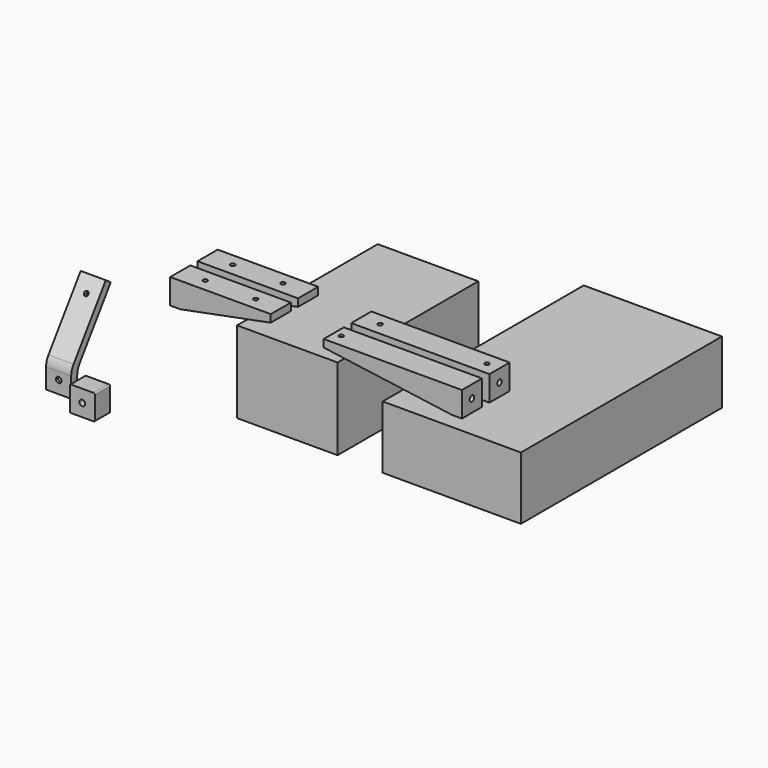
from build123d import *

# Parameters (mm, degrees)
F1_DEPTH   = 20
F3_R       = 1.75
F4_DEPTH   = 25
F5_R       = 3.5
F5_R_2     = 1.75
F6_DEPTH   = 3
F2_R       = 2.25
F7_DEPTH   = 25
F2_R_2     = 4
F8_DEPTH   = 4
F9_R       = 13
F10_W      = 80
F10_H      = 140
F11_DEPTH  = 65
F12_W      = 110
F12_H      = 200
F13_DEPTH  = 50
F15_DEPTH  = 20
F16_R      = 2.25
F17_DEPTH  = 122.8202211986
F18_DEPTH  = 4
F20_W      = 73.3484832836
F20_H      = 4
F22_R      = 1.75
F23_DEPTH  = 6.001
F22_R_2    = 3
F24_DEPTH  = 3
F26_DEPTH  = 20
F27_R      = 2.25
F28_DEPTH  = 4
F29_DEPTH  = 8.001
F31_W      = 102.9563014099
F31_H      = 4
F34_R      = 3
F34_R_2    = 1.75
F35_R      = 3
F35_R_2    = 1.75
F36_DEPTH  = 3
F36_FACE_R = 1.75
F37_DEPTH  = 9.6879868636
F38_DEPTH  = 3
F40_W      = 20
F40_H      = 20
F40_R      = 2.25
F41_DEPTH  = 15
F42_R      = 1


with BuildPart() as f1:
    # F0 (on Right) → F1 (new body)
    with BuildSketch(Plane.YZ):
        Polygon((0, 20), (0, 0), (6, 0), (6, 18.1082072667), (39.3294984468, 65.7076640392), (34.4145861811, 69.1491226573), align=None)
    extrude(amount=F1_DEPTH)

    # F3 (on face) → F4 (cut)
    with BuildSketch(Plane(origin=(0, -9.3969262079, 6.5797985667), x_dir=(1, 0, 0), z_dir=(0, -0.8191520443, 0.5735764364))):
        with Locations((10, 64.3830408858)):
            Circle(F3_R)
    extrude(amount=-F4_DEPTH, mode=Mode.SUBTRACT)

    # F5 (on face) → F6 (cut)
    with BuildSketch(Plane(origin=(0, -4.4820139421, 3.1383399486), x_dir=(-1, 0, 0), z_dir=(0, 0.8191520443, -0.5735764364))):
        with Locations((-10, 64.3830408858)):
            Circle(F5_R)
        with Locations((-10, 64.3830408858)):
            Circle(F5_R_2, mode=Mode.SUBTRACT)
    extrude(amount=-F6_DEPTH, mode=Mode.SUBTRACT)

    # F2 (on face) → F7 (cut)
    with BuildSketch(Plane(origin=(0, 6, 0), x_dir=(-1, 0, 0), z_dir=(0, 1, 0))):
        with Locations((-10, 10)):
            Circle(F2_R)
    extrude(amount=-F7_DEPTH, mode=Mode.SUBTRACT)

    # F2 (on face) → F8 (cut)
    with BuildSketch(Plane(origin=(0, 6, 0), x_dir=(-1, 0, 0), z_dir=(0, 1, 0))):
        with Locations((-10, 10)):
            Circle(F2_R_2)
        with Locations((-10, 10)):
            Circle(F2_R, mode=Mode.SUBTRACT)
    extrude(amount=-F8_DEPTH, mode=Mode.SUBTRACT)

    # F9
    f9_edges = [f1.edges().sort_by_distance(p)[0] for p in [
        (10, 6, 18.108207),
        (10, 0, 20),
    ]]
    fillet(f9_edges, radius=F9_R)


with BuildPart() as f11:
    # F10 (on Top) → F11 (new body)
    with BuildSketch(Plane.XY):
        with Locations((156.6803222895, 114.1342443228)):
            Rectangle(F10_W, F10_H)
    extrude(amount=F11_DEPTH)


with BuildPart() as f13:
    # F12 (on Top) → F13 (new body)
    with BuildSketch(Plane.XY):
        with Locations((288.3580553532, 143.2215481997)):
            Rectangle(F12_W, F12_H)
    extrude(amount=F13_DEPTH)


with BuildPart() as f15:
    # F14 (on Front) → F15 (new body)
    with BuildSketch(Plane.XZ):
        Polygon((114.8192211986, 124.3457761407), (114.8192211986, 104.3457761407), (122.8192211986, 104.3457761407), (122.8192211986, 118.3457761407), (194.8192211986, 118.3457761407), (194.8192211986, 124.3457761407), align=None)
    extrude(amount=F15_DEPTH)

    # F16 (on face) → F17 (cut, through all)
    with BuildSketch(Plane.YZ.offset(122.8192211986)):
        with Locations((-10, 114.3457761407)):
            Circle(F16_R)
    extrude(amount=-F17_DEPTH, mode=Mode.SUBTRACT)

    # F16 (on face) → F18 (cut)
    with BuildSketch(Plane.YZ.offset(122.8192211986)):
        with BuildLine():
            ThreePointArc((-10, 118.3457761407), (-12.8284271247, 111.5173490159), (-6, 114.3457761407))
            ThreePointArc((-6, 114.3457761407), (-7.1715728753, 117.1742032654), (-10, 118.3457761407))
        make_face()
        with Locations((-10, 114.3457761407)):
            Circle(F16_R, mode=Mode.SUBTRACT)
    extrude(amount=-F18_DEPTH, mode=Mode.SUBTRACT)

    # F20 (on 3pt) → F21 (join, up to the next surface of F15)
    with BuildSketch(Plane(origin=(-15.0758317834, 0, 77.532849172), x_dir=(0.9816153897, 0, 0.1908696591), z_dir=(-0.1908696591, 0, 0.9816153897))):
        with Locations((177.1519220381, -18)):
            Rectangle(F20_W, F20_H)
        with Locations((177.1519220381, -2)):
            Rectangle(F20_W, F20_H)
    extrude(until=Until.NEXT)

    # F22 (on face) → F23 (cut, through all)
    with BuildSketch(Plane(origin=(0, 0, 118.3457761407), x_dir=(1, 0, 0), z_dir=(0, 0, -1))):
        with Locations((134.8192211986, 10)):
            Circle(F22_R)
        with Locations((174.8192211986, 10)):
            Circle(F22_R)
    extrude(amount=-F23_DEPTH, mode=Mode.SUBTRACT)

    # F22 (on face) → F24 (cut)
    with BuildSketch(Plane(origin=(0, 0, 118.3457761407), x_dir=(1, 0, 0), z_dir=(0, 0, -1))):
        with Locations((134.8192211986, 10)):
            Circle(F22_R_2)
        with Locations((134.8192211986, 10)):
            Circle(F22_R, mode=Mode.SUBTRACT)
        with Locations((174.8192211986, 10)):
            Circle(F22_R_2)
        with Locations((174.8192211986, 10)):
            Circle(F22_R, mode=Mode.SUBTRACT)
    extrude(amount=-F24_DEPTH, mode=Mode.SUBTRACT)


with BuildPart() as f26:
    # F25 (on Front) → F26 (new body)
    with BuildSketch(Plane.XZ):
        Polygon((338.9809150696, 114.6587892771), (338.9809150696, 100.6587892771), (346.9809150696, 100.6587892771), (346.9809150696, 120.6587892771), (236.9809150696, 120.6587892771), (236.9809150696, 114.6587892771), align=None)
    extrude(amount=F26_DEPTH)

    # F27 (on face) → F28 (cut)
    with BuildSketch(Plane(origin=(338.9809150696, 0, 0), x_dir=(0, -1, 0), z_dir=(-1, 0, 0))):
        with BuildLine():
            ThreePointArc((10, 114.6587892771), (7.1715728753, 107.8303621523), (14, 110.6587892771))
            ThreePointArc((14, 110.6587892771), (12.8284271247, 113.4872164018), (10, 114.6587892771))
        make_face()
        with Locations((10, 110.6587892771)):
            Circle(F27_R, mode=Mode.SUBTRACT)
    extrude(amount=-F28_DEPTH, mode=Mode.SUBTRACT)

    # F29 (cut, through all): a face of the model
    f29_faces = [f26.faces().sort_by_distance(p)[0] for p in [
        (338.9809150696, -10, 110.6587892771),
    ]]
    extrude(f29_faces, amount=-F29_DEPTH, mode=Mode.SUBTRACT)

    # F31 (on 3pt) → F32 (join, up to the next surface of F26)
    with BuildSketch(Plane(origin=(19.8283972114, 0, 144.4640368262), x_dir=(0.9907115796, 0, -0.1359800207), z_dir=(0.1359800207, 0, 0.9907115796))):
        with Locations((270.6665828668, -18)):
            Rectangle(F31_W, F31_H)
        with Locations((270.6665828668, -2)):
            Rectangle(F31_W, F31_H)
    extrude(until=Until.NEXT)


with BuildPart() as f33_1:
    # F33: copy of F26
    add(f26.part.moved(Location((0, 27.4, 0))))


with BuildPart() as f36_tool:
    # F34 (on face) + F35 (on face) → F36 (new body)
    with BuildSketch(Plane(origin=(0, 0, 114.6587892771), x_dir=(1, 0, 0), z_dir=(0, 0, -1))):
        with Locations((242.9809150696, 10)):
            Circle(F34_R)
        with Locations((242.9809150696, 10)):
            Circle(F34_R_2, mode=Mode.SUBTRACT)
    with BuildSketch(Plane(origin=(0, 0, 114.6587892771), x_dir=(1, 0, 0), z_dir=(0, 0, -1))):
        with Locations((251.9809150696, -17.4)):
            Circle(F35_R)
        with Locations((251.9809150696, -17.4)):
            Circle(F35_R_2, mode=Mode.SUBTRACT)
        with BuildLine():
            Line((338.9809150696, -17.4), (338.9809150696, -15.1639320225))
            ThreePointArc((338.9809150696, -15.1639320225), (333.9809150696, -17.4), (338.9809150696, -19.6360679775))
            Line((338.9809150696, -19.6360679775), (338.9809150696, -17.4))
        make_face()
        with Locations((336.9809150696, -17.4)):
            Circle(F35_R_2, mode=Mode.SUBTRACT)
    extrude(amount=-F36_DEPTH)


with BuildPart() as f26_1:
    add(f26.part)

    # F36: cut by f36_tool
    add(f36_tool.part, mode=Mode.SUBTRACT)


with BuildPart() as f33_1_1:
    add(f33_1.part)

    # F36: cut by f36_tool
    add(f36_tool.part, mode=Mode.SUBTRACT)


with BuildPart() as f37_tool:
    # F36_face (on face) → F37 (new body, through all)
    with BuildSketch(Plane(origin=(242.9809150696, -10, 114.6587892771), x_dir=(1, 0, 0), z_dir=(0, 0, -1))):
        Circle(F36_FACE_R)
        with Locations((9, -27.4)):
            Circle(F36_FACE_R)
        with Locations((94, -27.4)):
            Circle(F36_FACE_R)
    extrude(amount=-F37_DEPTH)


with BuildPart() as f26_2:
    add(f26_1.part)

    # F37: cut by f37_tool
    add(f37_tool.part, mode=Mode.SUBTRACT)


with BuildPart() as f33_1_2:
    add(f33_1_1.part)

    # F37: cut by f37_tool
    add(f37_tool.part, mode=Mode.SUBTRACT)

    # F35 (on face) → F38 (cut, symmetric)
    with BuildSketch(Plane(origin=(0, 0, 114.6587892771), x_dir=(1, 0, 0), z_dir=(0, 0, -1))):
        with BuildLine():
            ThreePointArc((338.9809150696, -19.6360679775), (339.7195278571, -18.6247448714), (339.9809150696, -17.4))
            ThreePointArc((339.9809150696, -17.4), (339.7195278571, -16.1752551286), (338.9809150696, -15.1639320225))
            Line((338.9809150696, -15.1639320225), (338.9809150696, -17.4))
            Line((338.9809150696, -17.4), (338.9809150696, -19.6360679775))
        make_face()
    extrude(amount=F38_DEPTH, both=True, mode=Mode.SUBTRACT)


with BuildPart() as f39_1:
    # F39: copy of F15
    add(f15.part.moved(Location((0, 27.2, 0))))


with BuildPart() as f41:
    # F40 (on Front) → F41 (new body)
    with BuildSketch(Plane.XZ):
        with Locations((40.8435279876, 10)):
            Rectangle(F40_W, F40_H)
        with Locations((40.8435279876, 10)):
            Circle(F40_R, mode=Mode.SUBTRACT)
    extrude(amount=F41_DEPTH)

    # F42
    f42_edges = [f41.edges().sort_by_distance(p)[0] for p in [
        (50.843528, -7.5, 20),
        (50.843528, -7.5, 0),
        (30.843528, -7.5, 20),
        (30.843528, -7.5, 0),
    ]]
    fillet(f42_edges, radius=F42_R)


solid = Compound([f1.part, f11.part, f13.part, f15.part, f26_2.part, f33_1_2.part, f39_1.part, f41.part])
